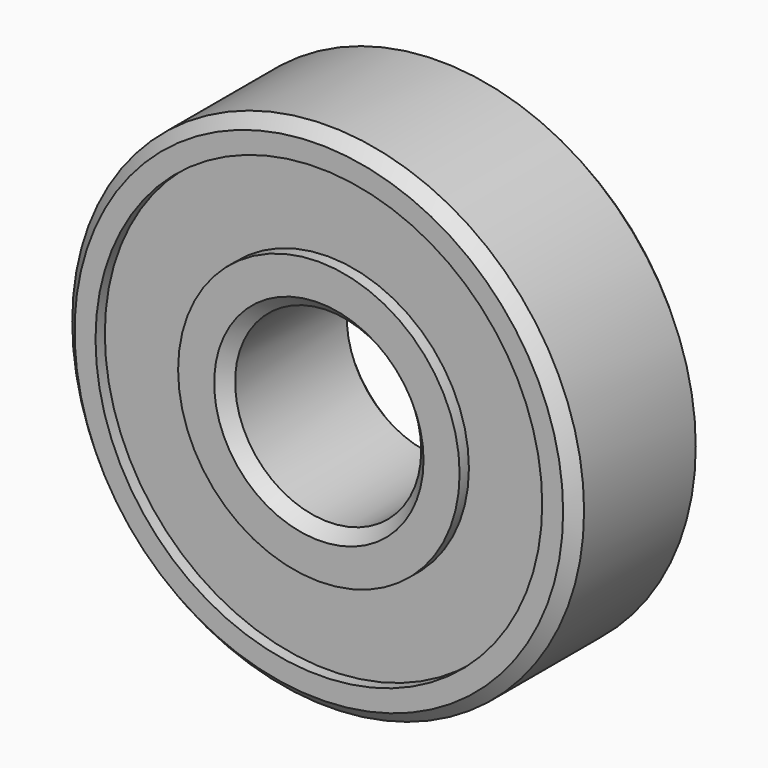
from build123d import *

# Parameters (mm, degrees)
F0_R          = 11
F0_R_2        = 4
F1_DEPTH      = 6
F2_R          = 11
F2_R_2        = 9.6
F2_R_3        = 6.05
F2_R_4        = 4
F3_DEPTH      = 0.5
F3_DEPTH_BACK = 6.5
F4_SIZE       = 0.49999


# Not quite as in the source:
# - a fillet or chamfer is up to 0.001 mm smaller than in the source, because OpenCascade refuses the exact size


with BuildPart() as f1:
    # F0 (on Front) → F1 (new body)
    with BuildSketch(Plane.XZ):
        Circle(F0_R)
        Circle(F0_R_2, mode=Mode.SUBTRACT)
    extrude(amount=-F1_DEPTH)

    # F2 (on face) → F3 (join, two sides)
    with BuildSketch(Plane.XZ) as f3_sk:
        Circle(F2_R)
        Circle(F2_R_2, mode=Mode.SUBTRACT)
        Circle(F2_R_3)
        Circle(F2_R_4, mode=Mode.SUBTRACT)
    extrude(amount=F3_DEPTH)
    extrude(f3_sk.sketch, amount=-F3_DEPTH_BACK)

    # F4 (size 0.5 in the source; OpenCascade refuses exactly that, so slightly less here)
    f4_edges = [f1.edges().sort_by_distance(p)[0] for p in [
        (-11, -0.5, 0),
        (-4, -0.5, 0),
        (-11, 6.5, 0),
        (-4, 6.5, 0),
    ]]
    chamfer(f4_edges, length=F4_SIZE)


solid = f1.part
